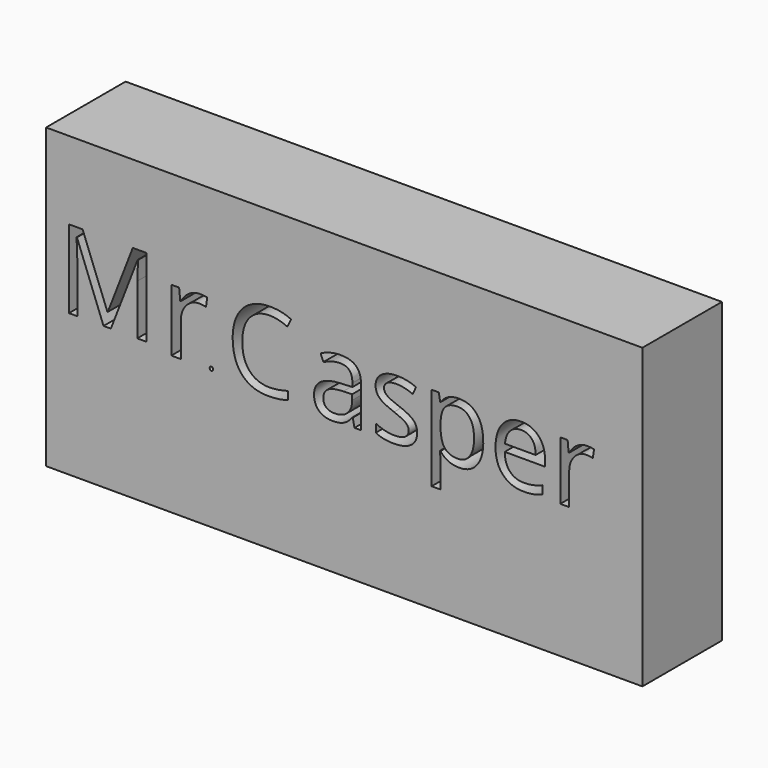
from build123d import *

# Parameters (mm, degrees)
F0_W           = 152.4
F0_H           = 76.2
F1_DEPTH       = 25.4
F2_TEXT_SIZE   = 28.0056510948
F2_TEXT_SIZE_2 = 27.6466107203
F2_TEXT_SIZE_3 = 29.8008891857
F2_TEXT_SIZE_4 = 28.0056562689
F2_TEXT_SIZE_5 = 7.1809316675
F3_DEPTH       = 12.7


# Not quite as in the source:
# - Text() gives the source's letters only with a copy of the font that has no kerning and outlines rounded to 1/6400 em; it was checked with that copy


with BuildPart() as f1:
    # F0 (on Front) → F1 (new body)
    with BuildSketch(Plane.XZ):
        with Locations((-0.603168043, 38.1)):
            Rectangle(F0_W, F0_H)
    extrude(amount=F1_DEPTH)

    # F2 (on face) → F3 (cut)
    with BuildSketch(Plane.XZ.offset(25.4)):
        with Locations((-73.7194865942, 36.3211818039)):
            Text('M', F2_TEXT_SIZE, font='Open Sans', text_align=(TextAlign.LEFT, TextAlign.BOTTOM))
        with Locations((-30.8062061667, 34.5115847886)):
            Text('C', F2_TEXT_SIZE_2, font='Open Sans', text_align=(TextAlign.LEFT, TextAlign.BOTTOM))
        with Locations((-47.3510846496, 35.2871268988)):
            Text('r', F2_TEXT_SIZE_3, font='Open Sans', text_align=(TextAlign.LEFT, TextAlign.BOTTOM))
        with Locations((-9.608078748, 34.2530682683)):
            Text('asper', F2_TEXT_SIZE_4, font='Open Sans', text_align=(TextAlign.LEFT, TextAlign.BOTTOM))
        with Locations((-35.5187501482, 35.2871268988)):
            Text('.', F2_TEXT_SIZE_5, font='Open Sans', text_align=(TextAlign.LEFT, TextAlign.BOTTOM))
    extrude(amount=-F3_DEPTH, mode=Mode.SUBTRACT)


solid = f1.part
